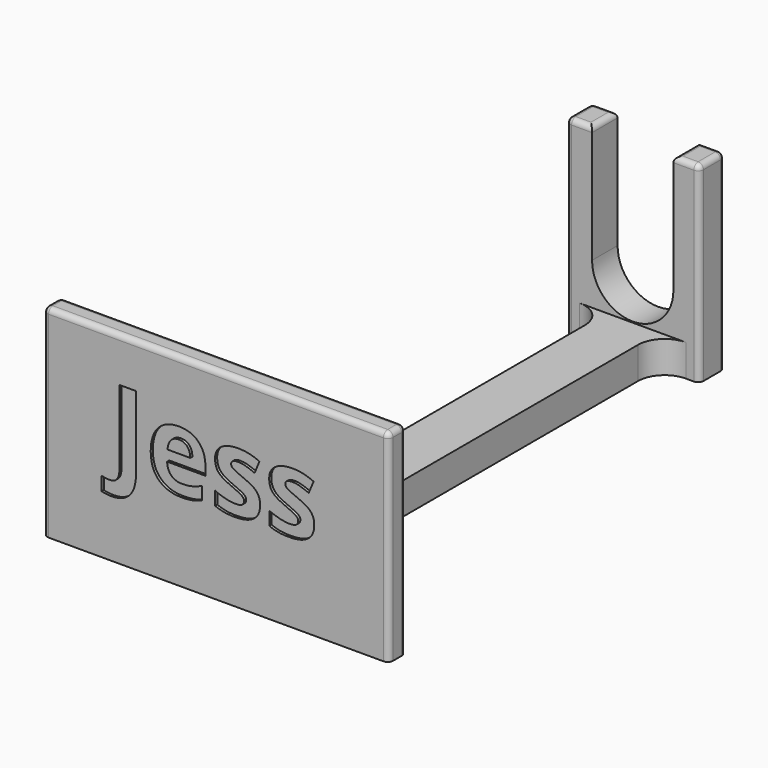
from build123d import *

# Parameters (mm, degrees)
F1_DEPTH      = 6
F3_DEPTH      = 32
F5_DEPTH      = 30
F7_DEPTH      = 6
F8_R          = 5
F9_R          = 5
F10_R         = 1
F11_TEXT_SIZE = 20.4898351209
F12_DEPTH     = 0.5


# Not quite as in the source:
# - Text() gives the source's letters only with a copy of the font that has no kerning and outlines rounded to 1/6400 em; it was checked with that copy


with BuildPart() as f1:
    # F0 (on Top) → F1 (new body)
    with BuildSketch(Plane.XY):
        Polygon((-32.5, -92), (-32.5, -96), (32.5, -96), (32.5, -92), (5, -92), (5, 2), (12.5, 2), (12.5, 8), (-12.5, 8), (-12.5, 2), (-5, 2), (-5, -92), align=None)
    extrude(amount=F1_DEPTH)

    # F2 (on face) → F3 (join)
    with BuildSketch(Plane.XY.offset(6)):
        Polygon((-5, -92), (-32.5, -92), (-32.5, -96), (32.5, -96), (32.5, -92), (5, -92), align=None)
    extrude(amount=F3_DEPTH)

    # F4 (on face) → F5 (join)
    with BuildSketch(Plane.XY.offset(6)):
        Polygon((12.5, 8), (-12.5, 8), (-12.5, 2), (-5, 2), (5, 2), (12.5, 2), align=None)
    extrude(amount=F5_DEPTH)

    # F6 (on face) → F7 (cut, through all)
    with BuildSketch(Plane(origin=(0, 8, 0), x_dir=(-1, 0, 0), z_dir=(0, 1, 0))):
        with BuildLine():
            ThreePointArc((-7.65, 13.85), (0, 21.5), (7.65, 13.85))
            Line((7.65, 13.85), (7.65, 36))
            Line((7.65, 36), (-7.65, 36))
            Line((-7.65, 36), (-7.65, 13.85))
        make_face()
        with BuildLine():
            ThreePointArc((-7.65, 13.85), (0, 6.2), (7.65, 13.85))
            ThreePointArc((7.65, 13.85), (0, 21.5), (-7.65, 13.85))
        make_face()
    extrude(amount=-F7_DEPTH, mode=Mode.SUBTRACT)

    # F8
    f8_edges = [f1.edges().sort_by_distance(p)[0] for p in [
        (-5, 2, 3),
        (5, 2, 3),
    ]]
    fillet(f8_edges, radius=F8_R)

    # F9
    f9_edges = [f1.edges().sort_by_distance(p)[0] for p in [
        (-5, -92, 3),
        (0, -92, 6),
        (5, -92, 3),
    ]]
    fillet(f9_edges, radius=F9_R)

    # F10
    f10_edges = [f1.edges().sort_by_distance(p)[0] for p in [
        (-7.65, 5, 36),
        (-10.075, 2, 36),
        (-12.5, 5, 36),
        (-10.075, 8, 36),
        (12.5, 5, 36),
        (10.075, 2, 36),
        (7.65, 5, 36),
        (10.075, 8, 36),
        (0, -92, 38),
        (-32.5, -94, 38),
        (0, -96, 38),
        (32.5, -94, 38),
        (32.5, -92, 19),
        (32.5, -96, 19),
        (12.5, 2, 18),
        (12.5, 8, 18),
        (-12.5, 8, 18),
        (-12.5, 2, 18),
        (-32.5, -96, 19),
        (-32.5, -92, 19),
    ]]
    fillet(f10_edges, radius=F10_R)

    # F11 (on face) → F12 (cut)
    with BuildSketch(Plane.XZ.offset(96)):
        with Locations((-20, 15)):
            Text('Jess', F11_TEXT_SIZE, font='Open Sans', font_style=FontStyle.BOLD, text_align=(TextAlign.LEFT, TextAlign.BOTTOM))
    extrude(amount=-F12_DEPTH, mode=Mode.SUBTRACT)


solid = f1.part
